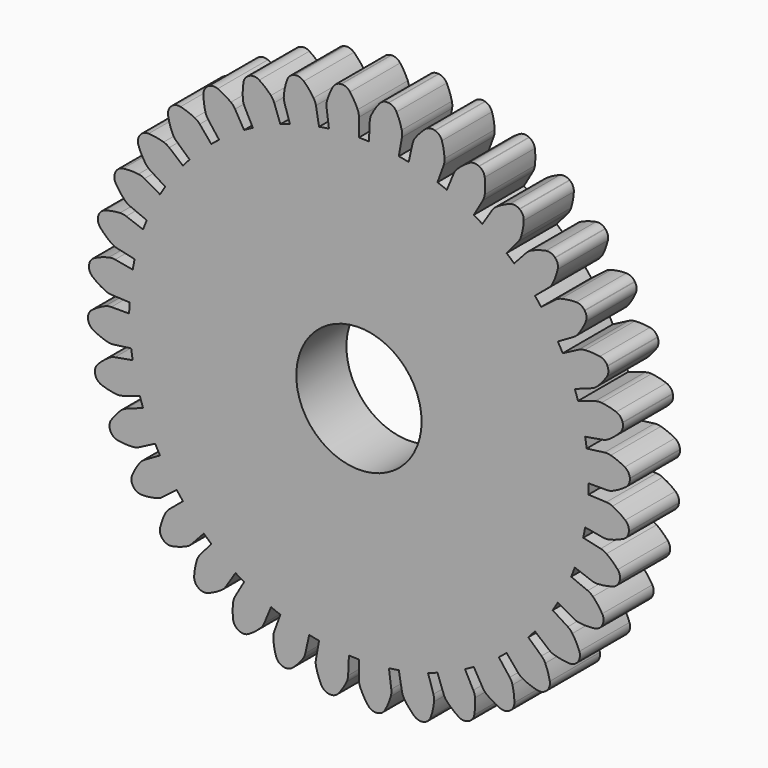
from build123d import *

# Parameters (mm, degrees)
F4_R     = 23.2791
F5_DEPTH = 6.35
F6_COUNT = 36
F8_R     = 6.35
F9_DEPTH = 6.3510001


with BuildPart() as f3:
    # F2 (on offset) → F3 section 0
    with BuildSketch(Plane.XZ.offset(6.35)):
        with BuildLine():
            ThreePointArc((-3.0385322813, 23.0799440724), (-1.5225259857, 23.22925766), (0, 23.2791))
            Line((0, 23.2791), (0, 25.0966573975))
            ThreePointArc((0, 25.0966573975), (-0.0325857473, 25.4179447998), (-0.1290158666, 25.7261471001))
            ThreePointArc((-0.1290158666, 25.7261471001), (-0.4746229855, 26.4149833331), (-0.9011320574, 27.0568786892))
            ThreePointArc((-0.9011320574, 27.0568786892), (-1.2889886908, 27.3681845534), (-1.7781282102, 27.4581102993))
            Line((-1.7781282102, 27.4581102993), (-1.7996073581, 27.4567024816))
            Line((-1.7996073581, 27.4567024816), (-1.821086506, 27.4552946639))
            ThreePointArc((-1.821086506, 27.4552946639), (-2.2943037038, 27.3022927262), (-2.638208601, 26.9430246774))
            ThreePointArc((-2.638208601, 26.9430246774), (-2.977284672, 26.2509502199), (-3.2300239035, 25.5228962951))
            ThreePointArc((-3.2300239035, 25.5228962951), (-3.285400577, 25.204744052), (-3.2757711275, 24.8819520144))
            Line((-3.2757711275, 24.8819520144), (-3.0385322813, 23.0799440724))
        make_face()
    # F0 (on Front) → F3 section 1
    with BuildSketch(Plane.XZ):
        with BuildLine():
            ThreePointArc((-3.0385322813, 23.0799440724), (-1.5225259857, 23.22925766), (0, 23.2791))
            Line((0, 23.2791), (0, 25.0966573975))
            ThreePointArc((0, 25.0966573975), (-0.0325857473, 25.4179447998), (-0.1290158666, 25.7261471001))
            ThreePointArc((-0.1290158666, 25.7261471001), (-0.4746229855, 26.4149833331), (-0.9011320574, 27.0568786892))
            ThreePointArc((-0.9011320574, 27.0568786892), (-1.2889886908, 27.3681845534), (-1.7781282102, 27.4581102993))
            Line((-1.7781282102, 27.4581102993), (-1.7996073581, 27.4567024816))
            Line((-1.7996073581, 27.4567024816), (-1.821086506, 27.4552946639))
            ThreePointArc((-1.821086506, 27.4552946639), (-2.2943037038, 27.3022927262), (-2.638208601, 26.9430246774))
            ThreePointArc((-2.638208601, 26.9430246774), (-2.977284672, 26.2509502199), (-3.2300239035, 25.5228962951))
            ThreePointArc((-3.2300239035, 25.5228962951), (-3.285400577, 25.204744052), (-3.2757711275, 24.8819520144))
            Line((-3.2757711275, 24.8819520144), (-3.0385322813, 23.0799440724))
        make_face()
    loft()

    # F4 (on offset) → F5 (join, through all)
    with BuildSketch(Plane.XZ.offset(6.35)):
        Circle(F4_R)
    extrude(amount=-F5_DEPTH)


with BuildPart() as f6_1:
    # F6: instance of F3
    add(f3.part.rotate(Axis((0, -6.35, 0), (0, -1, 0)), 1 * 360 / F6_COUNT))


with BuildPart() as f6_2:
    # F6: instance of F3
    add(f3.part.rotate(Axis((0, -6.35, 0), (0, -1, 0)), 2 * 360 / F6_COUNT))


with BuildPart() as f6_3:
    # F6: instance of F3
    add(f3.part.rotate(Axis((0, -6.35, 0), (0, -1, 0)), 3 * 360 / F6_COUNT))


with BuildPart() as f6_4:
    # F6: instance of F3
    add(f3.part.rotate(Axis((0, -6.35, 0), (0, -1, 0)), 4 * 360 / F6_COUNT))


with BuildPart() as f6_5:
    # F6: instance of F3
    add(f3.part.rotate(Axis((0, -6.35, 0), (0, -1, 0)), 5 * 360 / F6_COUNT))


with BuildPart() as f6_6:
    # F6: instance of F3
    add(f3.part.rotate(Axis((0, -6.35, 0), (0, -1, 0)), 6 * 360 / F6_COUNT))


with BuildPart() as f6_7:
    # F6: instance of F3
    add(f3.part.rotate(Axis((0, -6.35, 0), (0, -1, 0)), 7 * 360 / F6_COUNT))


with BuildPart() as f6_8:
    # F6: instance of F3
    add(f3.part.rotate(Axis((0, -6.35, 0), (0, -1, 0)), 8 * 360 / F6_COUNT))


with BuildPart() as f6_9:
    # F6: instance of F3
    add(f3.part.rotate(Axis((0, -6.35, 0), (0, -1, 0)), 9 * 360 / F6_COUNT))


with BuildPart() as f6_10:
    # F6: instance of F3
    add(f3.part.rotate(Axis((0, -6.35, 0), (0, -1, 0)), 10 * 360 / F6_COUNT))


with BuildPart() as f6_11:
    # F6: instance of F3
    add(f3.part.rotate(Axis((0, -6.35, 0), (0, -1, 0)), 11 * 360 / F6_COUNT))


with BuildPart() as f6_12:
    # F6: instance of F3
    add(f3.part.rotate(Axis((0, -6.35, 0), (0, -1, 0)), 12 * 360 / F6_COUNT))


with BuildPart() as f6_13:
    # F6: instance of F3
    add(f3.part.rotate(Axis((0, -6.35, 0), (0, -1, 0)), 13 * 360 / F6_COUNT))


with BuildPart() as f6_14:
    # F6: instance of F3
    add(f3.part.rotate(Axis((0, -6.35, 0), (0, -1, 0)), 14 * 360 / F6_COUNT))


with BuildPart() as f6_15:
    # F6: instance of F3
    add(f3.part.rotate(Axis((0, -6.35, 0), (0, -1, 0)), 15 * 360 / F6_COUNT))


with BuildPart() as f6_16:
    # F6: instance of F3
    add(f3.part.rotate(Axis((0, -6.35, 0), (0, -1, 0)), 16 * 360 / F6_COUNT))


with BuildPart() as f6_17:
    # F6: instance of F3
    add(f3.part.rotate(Axis((0, -6.35, 0), (0, -1, 0)), 17 * 360 / F6_COUNT))


with BuildPart() as f6_18:
    # F6: instance of F3
    add(f3.part.rotate(Axis((0, -6.35, 0), (0, -1, 0)), 18 * 360 / F6_COUNT))


with BuildPart() as f6_19:
    # F6: instance of F3
    add(f3.part.rotate(Axis((0, -6.35, 0), (0, -1, 0)), 19 * 360 / F6_COUNT))


with BuildPart() as f6_20:
    # F6: instance of F3
    add(f3.part.rotate(Axis((0, -6.35, 0), (0, -1, 0)), 20 * 360 / F6_COUNT))


with BuildPart() as f6_21:
    # F6: instance of F3
    add(f3.part.rotate(Axis((0, -6.35, 0), (0, -1, 0)), 21 * 360 / F6_COUNT))


with BuildPart() as f6_22:
    # F6: instance of F3
    add(f3.part.rotate(Axis((0, -6.35, 0), (0, -1, 0)), 22 * 360 / F6_COUNT))


with BuildPart() as f6_23:
    # F6: instance of F3
    add(f3.part.rotate(Axis((0, -6.35, 0), (0, -1, 0)), 23 * 360 / F6_COUNT))


with BuildPart() as f6_24:
    # F6: instance of F3
    add(f3.part.rotate(Axis((0, -6.35, 0), (0, -1, 0)), 24 * 360 / F6_COUNT))


with BuildPart() as f6_25:
    # F6: instance of F3
    add(f3.part.rotate(Axis((0, -6.35, 0), (0, -1, 0)), 25 * 360 / F6_COUNT))


with BuildPart() as f6_26:
    # F6: instance of F3
    add(f3.part.rotate(Axis((0, -6.35, 0), (0, -1, 0)), 26 * 360 / F6_COUNT))


with BuildPart() as f6_27:
    # F6: instance of F3
    add(f3.part.rotate(Axis((0, -6.35, 0), (0, -1, 0)), 27 * 360 / F6_COUNT))


with BuildPart() as f6_28:
    # F6: instance of F3
    add(f3.part.rotate(Axis((0, -6.35, 0), (0, -1, 0)), 28 * 360 / F6_COUNT))


with BuildPart() as f6_29:
    # F6: instance of F3
    add(f3.part.rotate(Axis((0, -6.35, 0), (0, -1, 0)), 29 * 360 / F6_COUNT))


with BuildPart() as f6_30:
    # F6: instance of F3
    add(f3.part.rotate(Axis((0, -6.35, 0), (0, -1, 0)), 30 * 360 / F6_COUNT))


with BuildPart() as f6_31:
    # F6: instance of F3
    add(f3.part.rotate(Axis((0, -6.35, 0), (0, -1, 0)), 31 * 360 / F6_COUNT))


with BuildPart() as f6_32:
    # F6: instance of F3
    add(f3.part.rotate(Axis((0, -6.35, 0), (0, -1, 0)), 32 * 360 / F6_COUNT))


with BuildPart() as f6_33:
    # F6: instance of F3
    add(f3.part.rotate(Axis((0, -6.35, 0), (0, -1, 0)), 33 * 360 / F6_COUNT))


with BuildPart() as f6_34:
    # F6: instance of F3
    add(f3.part.rotate(Axis((0, -6.35, 0), (0, -1, 0)), 34 * 360 / F6_COUNT))


with BuildPart() as f6_35:
    # F6: instance of F3
    add(f3.part.rotate(Axis((0, -6.35, 0), (0, -1, 0)), 35 * 360 / F6_COUNT))


with BuildPart() as f6_31_1:
    add(f6_31.part)

    # F7: union F6_2, F3, F6_1, F6_35, F6_34, F6_33, F6_32, F6_30, F6_29, F6_28, F6_27, F6_26, F6_25, F6_24, F6_23, F6_22, F6_21, F6_20, F6_19, F6_18, F6_17, F6_16, F6_15, F6_14, F6_13, F6_12, F6_11, F6_10, F6_9, F6_8, F6_7, F6_6, F6_5, F6_4, F6_3
    add(f6_2.part)
    add(f3.part)
    add(f6_1.part)
    add(f6_35.part)
    add(f6_34.part)
    add(f6_33.part)
    add(f6_32.part)
    add(f6_30.part)
    add(f6_29.part)
    add(f6_28.part)
    add(f6_27.part)
    add(f6_26.part)
    add(f6_25.part)
    add(f6_24.part)
    add(f6_23.part)
    add(f6_22.part)
    add(f6_21.part)
    add(f6_20.part)
    add(f6_19.part)
    add(f6_18.part)
    add(f6_17.part)
    add(f6_16.part)
    add(f6_15.part)
    add(f6_14.part)
    add(f6_13.part)
    add(f6_12.part)
    add(f6_11.part)
    add(f6_10.part)
    add(f6_9.part)
    add(f6_8.part)
    add(f6_7.part)
    add(f6_6.part)
    add(f6_5.part)
    add(f6_4.part)
    add(f6_3.part)

    # F8 (on face) → F9 (cut, through all)
    with BuildSketch(Plane.XZ.offset(6.35)):
        Circle(F8_R)
    extrude(amount=-F9_DEPTH, mode=Mode.SUBTRACT)


solid = f6_31_1.part
